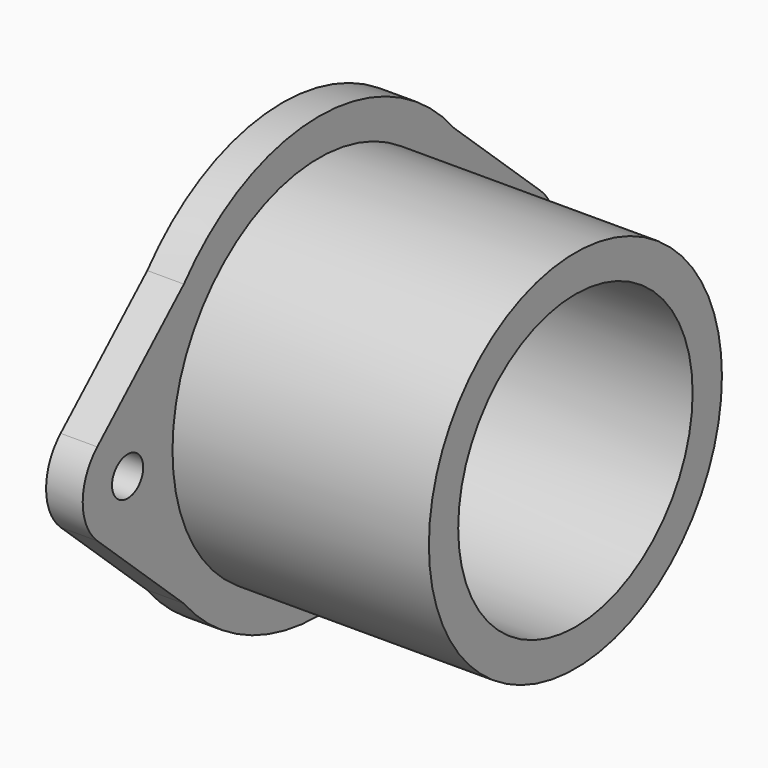
from build123d import *

# Parameters (mm, degrees)
F0_R     = 31.75
F0_R_2   = 25.4
F1_DEPTH = 50.8
F0_R_3   = 3.3782
F2_DEPTH = 6.35


# Not quite as in the source:
# - a feature names something its author has since deleted; it is built from what else it names


with BuildPart() as f1:
    # F0 (on Right) → F1 (new body)
    with BuildSketch(Plane.YZ):
        Circle(F0_R)
        Circle(F0_R_2, mode=Mode.SUBTRACT)
    extrude(amount=F1_DEPTH)

    # F0 (on Right) → F2 (join)
    with BuildSketch(Plane.YZ):
        with BuildLine():
            Line((-48.0517219843, -7.1712400574), (-29.2791039707, -24.3791728874))
            ThreePointArc((-29.2791039707, -24.3791728874), (0, -38.1), (29.2791039707, -24.3791728874))
            Line((29.2791039707, -24.3791728874), (48.0517219843, -7.1712400574))
            ThreePointArc((48.0517219843, -7.1712400574), (51.2064, 0), (48.0517219843, 7.1712400574))
            Line((48.0517219843, 7.1712400574), (29.2791039707, 24.3791728874))
            ThreePointArc((29.2791039707, 24.3791728874), (0, 38.1), (-29.2791039707, 24.3791728874))
            Line((-29.2791039707, 24.3791728874), (-48.0517219843, 7.1712400574))
            ThreePointArc((-48.0517219843, 7.1712400574), (-51.2064, 0), (-48.0517219843, -7.1712400574))
        make_face()
        with Locations((-41.4782, 0)):
            Circle(F0_R_3, mode=Mode.SUBTRACT)
        Circle(F0_R, mode=Mode.SUBTRACT)
        with Locations((41.4782, 0)):
            Circle(F0_R_3, mode=Mode.SUBTRACT)
    extrude(amount=F2_DEPTH)


solid = f1.part
